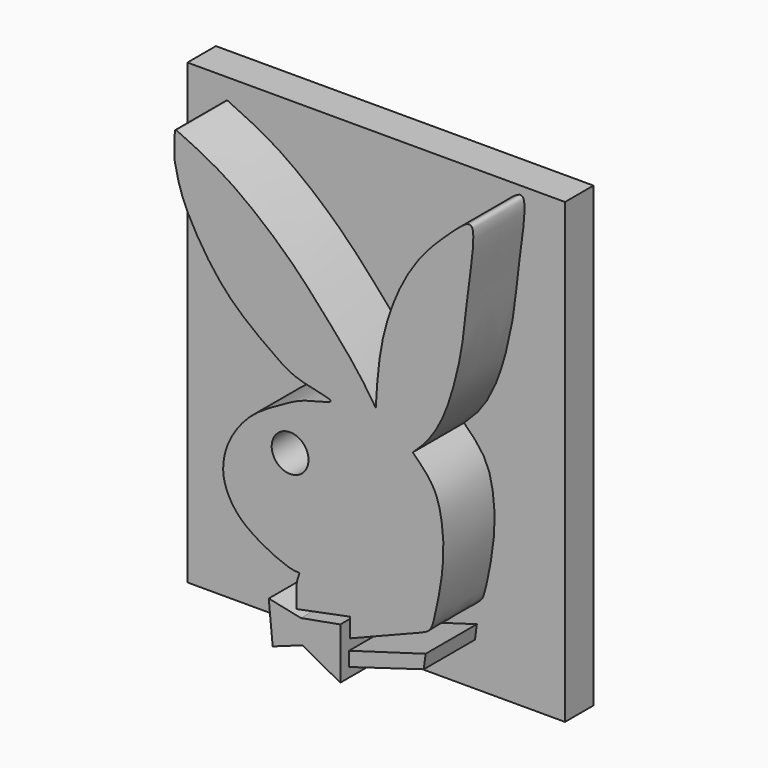
from build123d import *

# Parameters (mm, degrees)
F0_R     = 2.5881190518
F1_DEPTH = 14
F2_W     = 53.0733359046
F2_H     = 64.3425136805
F3_DEPTH = 5


# Not quite as in the source:
# - a feature names something its author has since deleted; it is built from what else it names


with BuildPart() as f1:
    # F0 (on Front) → F1 (new body)
    with BuildSketch(Plane.XZ):
        with BuildLine():
            add(Edge.make_bspline(
                [(-44.3972833455, 61.4496953785), (-44.4490464675, 61.4568435425), (-44.565056792, 61.4728638439), (-44.681468286, 61.2009254932), (-44.6765757123, 58.4695911448), (-44.658618745, 57.8367841289), (-44.6519888937, 57.6031468809)],
                knots=[0, 0, 0, 0, 0.1083960468, 0.2429347395, 0.7204856463, 1, 1, 1, 1], degree=3))
            add(Edge.make_bspline(
                [(-44.6519888937, 57.6031468809), (-44.4003246793, 56.3541446109), (-43.8473826271, 53.6099090822), (-41.126808261, 48.4869449794), (-36.9683037207, 42.6682303212), (-30.5102740969, 37.9993132704), (-27.5245233409, 35.9740625461), (-20.6501644663, 35.0472789539), (-26.5215643921, 34.07988225), (-29.4570014209, 32.3971668125), (-34.1239486196, 29.8359159403), (-36.8205871097, 26.084209941), (-37.7045777644, 23.5983639301), (-38.0421931941, 20.7389531569), (-36.5846802801, 17.270299258), (-33.3696698148, 14.4627164238), (-28.2588031256, 12.1527927032), (-26.9118321529, 12.4074409024), (-27.6583389074, 11.2686028265), (-27.5666216616, 9.1459115136), (-27.5041740388, 7.7006323263)],
                knots=[0, 0, 0, 0, 0.0559294052, 0.1228848533, 0.1993895751, 0.2771236427, 0.3355004813, 0.3929729537, 0.4441332892, 0.5005835066, 0.5646576506, 0.6244890061, 0.669608993, 0.7160670006, 0.7687175891, 0.8285841882, 0.8948534111, 0.9199839904, 0.9455194108, 1, 1, 1, 1], degree=3))
            add(Edge.make_bspline(
                [(-27.5041740388, 7.7006323263), (-26.3024494279, 7.9527125617), (-23.8619408464, 8.4646468037), (-21.2983337476, 8.9537756253), (-19.9970658869, 9.2020537704)],
                knots=[0, 0, 0, 0, 0.4924074514, 1, 1, 1, 1], degree=3))
            add(Edge.make_bspline(
                [(-19.9970658869, 9.2020537704), (-19.9970658869, 8.3064689922), (-19.9970658869, 7.4108842139), (-19.9970658869, 6.5152994357)],
                knots=[0, 0, 0, 0, 2.6867543347, 2.6867543347, 2.6867543347, 2.6867543347], degree=3))
            add(Edge.make_bspline(
                [(-19.9970658869, 6.5152994357), (-16.0512076561, 8.0698825341), (-10.5172081741, 10.2501590564), (-8.5887342269, 11.0811763191), (-7.9460625464, 13.6378911094), (-6.6753789765, 19.9029977792), (-6.9843010939, 25.2696178352), (-8.0572100828, 29.3332570636), (-10.1306055922, 31.3622079575), (-11.1860912293, 32.3950685561)],
                knots=[0, 0, 0, 0, 0.2156238193, 0.3024087624, 0.4033101833, 0.5728250723, 0.7293840486, 0.8622398628, 1, 1, 1, 1], degree=3))
            add(Edge.make_bspline(
                [(-11.1860912293, 32.3950685561), (-10.5212378252, 33.0107248909), (-9.0471212528, 34.3801242718), (-6.3090018579, 38.6642251737), (-4.0541052944, 47.6794637923), (-3.679815117, 53.9321618248), (-2.2206591136, 62.6908933724), (-3.4427635635, 63.4443985763), (-5.3796876825, 61.7439260973), (-7.032660786, 60.2214249236), (-10.2555515002, 56.9987891103), (-13.4853950363, 51.7094244106), (-15.9017235257, 44.2992201365), (-16.2172110494, 39.0461386917), (-16.3931064308, 36.2177453935)],
                knots=[0, 0, 0, 0, 0.0625353907, 0.146564244, 0.2594282324, 0.3614765557, 0.4683826109, 0.5006173225, 0.5572565569, 0.6156302084, 0.694103097, 0.7881892855, 0.8925081532, 1, 1, 1, 1], degree=3))
            add(Edge.make_bspline(
                [(-16.3931064308, 36.2177453935), (-17.187345901, 37.4388284437), (-18.9834532323, 40.2002074745), (-24.0747269617, 45.9440130974), (-28.5123048659, 50.9302417978), (-36.8587882285, 57.9637418804), (-41.9903191322, 60.3366661613), (-44.3972833455, 61.4496953785)],
                knots=[0, 0, 0, 0, 0.1581257064, 0.3575882981, 0.5504459332, 0.7891349441, 1, 1, 1, 1], degree=3))
        make_face()
        with Locations((-28.4292511642, 26.7006196082)):
            Circle(F0_R, mode=Mode.SUBTRACT)
    extrude(amount=F1_DEPTH)


with BuildPart() as f1b:
    # F0 (on Front) → F1, piece 2 (new body)
    with BuildSketch(Plane.XZ):
        Polygon((-26.9076004624, 6.7828586325), (-31.4336456358, 7.7327694744), (-30.8748763055, 1.9774257671), (-26.6840923578, 3.4861082677), (-21.3757641613, 0.5804976099), (-21.3757641613, 7.7886469662), align=None)
    extrude(amount=F1_DEPTH)


with BuildPart() as f1c:
    # F0 (on Front) → F1, piece 3 (new body)
    with BuildSketch(Plane.XZ):
        Polygon((-9.3785477802, 8.0618355423), (-20.1464686543, 4.9389135092), (-20.1464686543, 2.9273370747), (-9.6415681764, 6.0564558953), align=None)
    extrude(amount=F1_DEPTH)


with BuildPart() as f3:
    # F2 (on Front) → F3 (new body)
    with BuildSketch(Plane.XZ):
        with Locations((-23.5232871491, 32.1712568402)):
            Rectangle(F2_W, F2_H)
    extrude(amount=F3_DEPTH)


solid = Compound([f1.part, f1b.part, f1c.part, f3.part])
